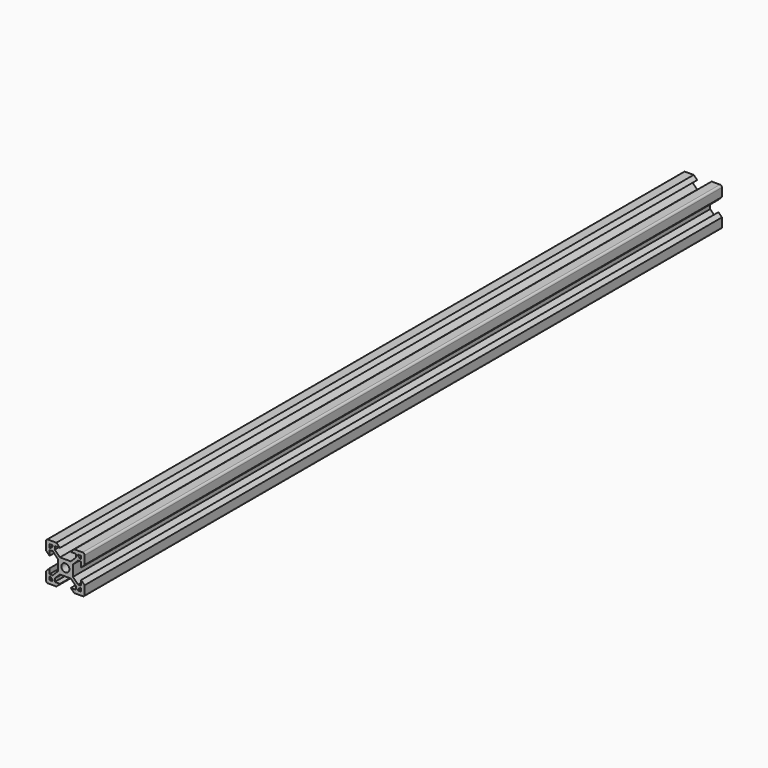
from build123d import *

# Parameters (mm, degrees)
F0_W            = 20
F0_H            = 20
F1_DEPTH        = 413
F2_R            = 2.1
F3_DEPTH        = 413.001
F4_R            = 1
F6_DEPTH        = 413.001
F6_COPIES_COUNT = 4


# Not quite as in the source:
# - a pattern or mirror of a feature is missing from the dataset's text; its kind, count and spacing are read off the source's solid


with BuildPart() as f1:
    # F0 (on Front) → F1 (new body)
    with BuildSketch(Plane.XZ):
        Rectangle(F0_W, F0_H)
    extrude(amount=F1_DEPTH)

    # F2 (on face) → F3 (cut, through all)
    with BuildSketch(Plane.XZ.offset(413)):
        Circle(F2_R)
    extrude(amount=-F3_DEPTH, mode=Mode.SUBTRACT)

    # F4
    f4_edges = [f1.edges().sort_by_distance(p)[0] for p in [
        (-10, -206.5, 10),
        (10, -206.5, 10),
        (10, -206.5, -10),
        (-10, -206.5, -10),
    ]]
    fillet(f4_edges, radius=F4_R)

    # F5 (on face) → F6 (cut, through all)
    with BuildSketch(Plane.XZ.offset(413)):
        Polygon((0, 3.9006601718), (0, 10), (-2.84, 10), (-4.64, 10), (-2.84, 8.2), (-5.4993398282, 8.2), (-5.4993398282, 6.56), (-2.84, 3.9006601718), align=None)
        Polygon((-6.5693398282, 8.2), (-8.2, 8.2), (-7.0953059148, 7.0953059148), (-6.5693398282, 7.6212720014), align=None)
    f6 = extrude(amount=-F6_DEPTH, mode=Mode.SUBTRACT)

    # F6_copies: F6 ×4 about axis
    f6_copies_axis = Axis((0, 0, 0), (0, 1, 0))
    for i in range(1, F6_COPIES_COUNT):
        add(f6.rotate(f6_copies_axis, i * 360 / F6_COPIES_COUNT), mode=Mode.SUBTRACT)

    # F6_copies1: F6 across plane
    add(f6.mirror(Plane(origin=(0, 0, 0), x_dir=(-0.7071067812, 0, -0.7071067812), z_dir=(0.7071067812, 0, -0.7071067812))), mode=Mode.SUBTRACT)

    # F6_copies2: F6 across plane
    add(f6.mirror(Plane(origin=(0, 0, 0), x_dir=(-1, 0, 0), z_dir=(0, 0, -1))), mode=Mode.SUBTRACT)

    # F6_copies3: F6 across plane
    add(f6.mirror(Plane(origin=(0, 0, 0), x_dir=(0, 0, 1), z_dir=(1, 0, 0))), mode=Mode.SUBTRACT)

    # F6_copies4: F6 across plane
    add(f6.mirror(Plane(origin=(0, 0, 0), x_dir=(0.7071067812, 0, -0.7071067812), z_dir=(-0.7071067812, 0, -0.7071067812))), mode=Mode.SUBTRACT)


solid = f1.part
